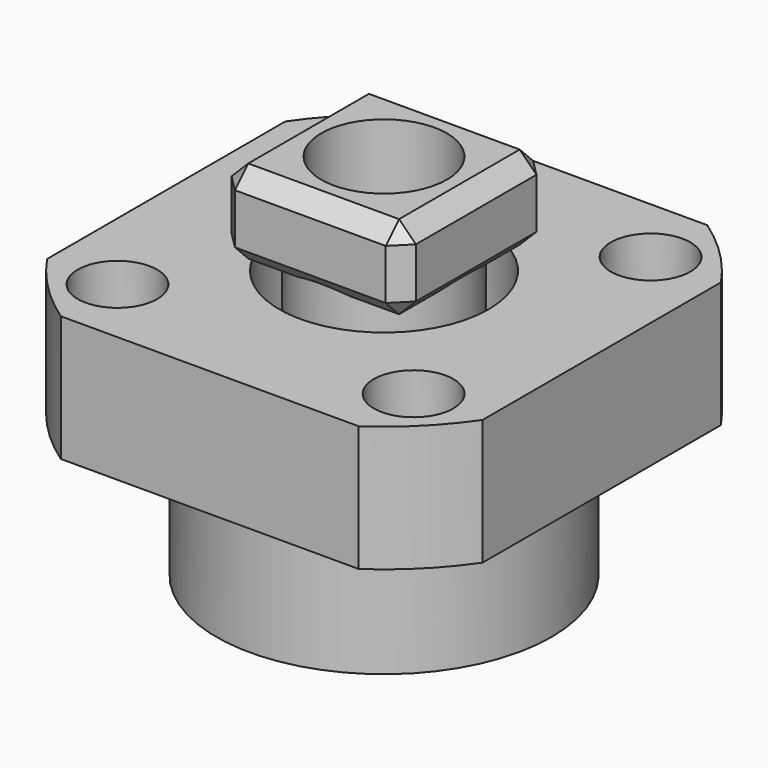
from build123d import *

# Parameters (mm, degrees)
F0_R            = 20
F1_DEPTH        = 17
F3_DEPTH        = 15
F4_R            = 12.5
F4_R_2          = 9.5
F5_DEPTH        = 10
F6_R            = 9.5
F7_DEPTH        = 2
F8_W            = 22
F8_H            = 22
F9_DEPTH        = 10
F10_T1_DEPTH    = 2.5403411844
F10_T3_DEPTH    = 2.5403411844
F10_T5_DEPTH    = 2.5403411844
F10_T7_DEPTH    = 2.5403411844
F10_T9_DEPTH    = 2.5403411844
F10_T11_DEPTH   = 2.5403411844
F10_T13_DEPTH   = 2.5403411844
F10_T15_DEPTH   = 2.5403411844
F10_T17_DEPTH   = 32.2867319519
F10_T19_DEPTH   = 32.2867319519
F10_T24_DEPTH   = 20.2867319519
F10_T29_DEPTH   = 20.2867319519
F10_T34_DEPTH   = 20.2867319519
F10_T39_DEPTH   = 20.2867319519
F10_T44_DEPTH   = 32.2867319519
F10_S45_R       = 9.5
F10_T46_DEPTH   = 18
F10_T50_DEPTH   = 32.2867319519
F10_S51_R       = 9.5
F10_T52_DEPTH   = 18
F10_T56_DEPTH   = 32.2867319519
F10_S57_R       = 9.5
F10_T58_DEPTH   = 18
F10_T62_DEPTH   = 32.2867319519
F10_S63_R       = 9.5
F10_T64_DEPTH   = 18
F11_R           = 10
F12_DEPTH       = 5
F13_R           = 7.5
F14_DEPTH       = 44.001
F16_D           = 5.5
F16_CBORE_D     = 9.5
F16_CBORE_DEPTH = 5


# Not quite as in the source:
# - a fillet or chamfer that OpenCascade refuses, or shapes differently, is made with other operations: its cross-section is extruded or revolved along the edge and cut away or added


with BuildPart() as f1:
    # F0 (on Top) → F1 (new body)
    with BuildSketch(Plane.XY):
        Circle(F0_R)
    extrude(amount=-F1_DEPTH)

    # F2 (on Top) → F3 (join)
    with BuildSketch(Plane.XY):
        with BuildLine():
            Line((17.7834192438, 26), (-17.7834192438, 26))
            ThreePointArc((-17.7834192438, 26), (-22.2738636074, 22.2738636074), (-26, 17.7834192438))
            Line((-26, 17.7834192438), (-26, -17.7834192438))
            ThreePointArc((-26, -17.7834192438), (-22.2738636074, -22.2738636074), (-17.7834192438, -26))
            Line((-17.7834192438, -26), (17.7834192438, -26))
            ThreePointArc((17.7834192438, -26), (22.2738636074, -22.2738636074), (26, -17.7834192438))
            Line((26, -17.7834192438), (26, 17.7834192438))
            ThreePointArc((26, 17.7834192438), (22.2738636074, 22.2738636074), (17.7834192438, 26))
        make_face()
    extrude(amount=F3_DEPTH)

    # F4 (on face) → F5 (cut)
    with BuildSketch(Plane.XY.offset(15)):
        Circle(F4_R)
        Circle(F4_R_2, mode=Mode.SUBTRACT)
    extrude(amount=-F5_DEPTH, mode=Mode.SUBTRACT)

    # F6 (on face) → F7 (join)
    with BuildSketch(Plane.XY.offset(15)):
        Circle(F6_R)
    extrude(amount=F7_DEPTH)

    # F8 (on face) → F9 (join)
    with BuildSketch(Plane.XY.offset(17)):
        Rectangle(F8_W, F8_H)
    extrude(amount=F9_DEPTH)

    # F10: chamfer of 2 on 12 edges, made by hand

    # F10_s2 → F10_t1 (cut)
    with BuildSketch(Plane(origin=(-0.3333333333, 0.3333333333, -0.3333333333), x_dir=(-0.7071067812, -0.7071067812, 0), z_dir=(-0.5773502692, 0.5773502692, -0.5773502692))):
        Polygon((-1.4142135624, 23.6784008469), (1.4142135624, 23.6784008469), (0, 21.2289111041), align=None)
    extrude(amount=F10_T1_DEPTH, mode=Mode.SUBTRACT)

    # F10_s4 → F10_t3 (cut)
    with BuildSketch(Plane(origin=(-15, 15, 15), x_dir=(-0.7071067812, -0.7071067812, 0), z_dir=(-0.5773502692, 0.5773502692, 0.5773502692))):
        Polygon((-1.4142135624, 12.2474487139), (1.4142135624, 12.2474487139), (0, 14.6969384567), align=None)
    extrude(amount=F10_T3_DEPTH, mode=Mode.SUBTRACT)

    # F10_s6 → F10_t5 (cut)
    with BuildSketch(Plane(origin=(0.3333333333, 0.3333333333, -0.3333333333), x_dir=(-0.7071067812, 0.7071067812, 0), z_dir=(0.5773502692, 0.5773502692, -0.5773502692))):
        Polygon((1.4142135624, 23.6784008469), (-1.4142135624, 23.6784008469), (0, 21.2289111041), align=None)
    extrude(amount=F10_T5_DEPTH, mode=Mode.SUBTRACT)

    # F10_s8 → F10_t7 (cut)
    with BuildSketch(Plane(origin=(15, 15, 15), x_dir=(-0.7071067812, 0.7071067812, 0), z_dir=(0.5773502692, 0.5773502692, 0.5773502692))):
        Polygon((1.4142135624, 12.2474487139), (-1.4142135624, 12.2474487139), (0, 14.6969384567), align=None)
    extrude(amount=F10_T7_DEPTH, mode=Mode.SUBTRACT)

    # F10_s10 → F10_t9 (cut)
    with BuildSketch(Plane(origin=(0.3333333333, -0.3333333333, -0.3333333333), x_dir=(0.7071067812, 0.7071067812, 0), z_dir=(0.5773502692, -0.5773502692, -0.5773502692))):
        Polygon((1.4142135624, 23.6784008469), (0, 21.2289111041), (-1.4142135624, 23.6784008469), align=None)
    extrude(amount=F10_T9_DEPTH, mode=Mode.SUBTRACT)

    # F10_s12 → F10_t11 (cut)
    with BuildSketch(Plane(origin=(15, -15, 15), x_dir=(0.7071067812, 0.7071067812, 0), z_dir=(0.5773502692, -0.5773502692, 0.5773502692))):
        Polygon((1.4142135624, 12.2474487139), (0, 14.6969384567), (-1.4142135624, 12.2474487139), align=None)
    extrude(amount=F10_T11_DEPTH, mode=Mode.SUBTRACT)

    # F10_s14 → F10_t13 (cut)
    with BuildSketch(Plane(origin=(-0.3333333333, -0.3333333333, -0.3333333333), x_dir=(0.7071067812, -0.7071067812, 0), z_dir=(-0.5773502692, -0.5773502692, -0.5773502692))):
        Polygon((-1.4142135624, 23.6784008469), (0, 21.2289111041), (1.4142135624, 23.6784008469), align=None)
    extrude(amount=F10_T13_DEPTH, mode=Mode.SUBTRACT)

    # F10_s16 → F10_t15 (cut)
    with BuildSketch(Plane(origin=(-15, -15, 15), x_dir=(0.7071067812, -0.7071067812, 0), z_dir=(-0.5773502692, -0.5773502692, 0.5773502692))):
        Polygon((-1.4142135624, 12.2474487139), (0, 14.6969384567), (1.4142135624, 12.2474487139), align=None)
    extrude(amount=F10_T15_DEPTH, mode=Mode.SUBTRACT)

    # F10_s18 → F10_t17 (cut)
    with BuildSketch(Plane.XZ.offset(-16.1433659759)):
        Polygon((-11, 25), (-9, 27), (-11, 27), align=None)
        Polygon((11, 25), (9, 27), (11, 27), align=None)
    extrude(amount=F10_T17_DEPTH, mode=Mode.SUBTRACT)

    # F10_s20 → F10_t19 (cut)
    with BuildSketch(Plane.YZ.offset(-16.1433659759)):
        Polygon((-9, 27), (-11, 25), (-11, 27), align=None)
        Polygon((11, 25), (9, 27), (11, 27), align=None)
    extrude(amount=F10_T19_DEPTH, mode=Mode.SUBTRACT)


with BuildPart() as f10_tool22:
    # F10_s23 → F10_t24 (new body)
    with BuildSketch(Plane.XY.offset(11.8566340241)):
        Polygon((-9, 11), (-11, 9), (-11, 11), align=None)
    extrude(amount=F10_T24_DEPTH)

    split(bisect_by=Plane.XY.offset(15), keep=Keep.TOP)


with BuildPart() as f1_1:
    add(f1.part)

    # F10_t21: cut F10_tool22
    add(f10_tool22.part, mode=Mode.SUBTRACT)


with BuildPart() as f10_tool27:
    # F10_s28 → F10_t29 (new body)
    with BuildSketch(Plane.XY.offset(11.8566340241)):
        Polygon((9, 11), (11, 9), (11, 11), align=None)
    extrude(amount=F10_T29_DEPTH)

    split(bisect_by=Plane.XY.offset(15), keep=Keep.TOP)


with BuildPart() as f1_2:
    add(f1_1.part)

    # F10_t26: cut F10_tool27
    add(f10_tool27.part, mode=Mode.SUBTRACT)


with BuildPart() as f10_tool32:
    # F10_s33 → F10_t34 (new body)
    with BuildSketch(Plane.XY.offset(11.8566340241)):
        Polygon((11, -9), (9, -11), (11, -11), align=None)
    extrude(amount=F10_T34_DEPTH)

    split(bisect_by=Plane.XY.offset(15), keep=Keep.TOP)


with BuildPart() as f1_3:
    add(f1_2.part)

    # F10_t31: cut F10_tool32
    add(f10_tool32.part, mode=Mode.SUBTRACT)


with BuildPart() as f10_tool37:
    # F10_s38 → F10_t39 (new body)
    with BuildSketch(Plane.XY.offset(11.8566340241)):
        Polygon((-11, -9), (-9, -11), (-11, -11), align=None)
    extrude(amount=F10_T39_DEPTH)

    split(bisect_by=Plane.XY.offset(15), keep=Keep.TOP)


with BuildPart() as f1_4:
    add(f1_3.part)

    # F10_t36: cut F10_tool37
    add(f10_tool37.part, mode=Mode.SUBTRACT)


with BuildPart() as f10_tool42:
    # F10_s43 → F10_t44 (new body)
    with BuildSketch(Plane.XZ.offset(-16.1433659759)):
        Polygon((-11, 19), (-9, 17), (-11, 17), align=None)
    extrude(amount=F10_T44_DEPTH)

    # F10_s45 → F10_t46 (cut, symmetric)
    with BuildSketch(Plane.XY.offset(18)):
        Circle(F10_S45_R)
    extrude(amount=F10_T46_DEPTH, both=True, mode=Mode.SUBTRACT)


with BuildPart() as f1_5:
    add(f1_4.part)

    # F10_t41: cut F10_tool42
    add(f10_tool42.part, mode=Mode.SUBTRACT)


with BuildPart() as f10_tool48:
    # F10_s49 → F10_t50 (new body)
    with BuildSketch(Plane.XZ.offset(16.1433659759)):
        Polygon((11, 19), (9, 17), (11, 17), align=None)
    extrude(amount=-F10_T50_DEPTH)

    # F10_s51 → F10_t52 (cut, symmetric)
    with BuildSketch(Plane.XY.offset(18)):
        Circle(F10_S51_R)
    extrude(amount=F10_T52_DEPTH, both=True, mode=Mode.SUBTRACT)


with BuildPart() as f1_6:
    add(f1_5.part)

    # F10_t47: cut F10_tool48
    add(f10_tool48.part, mode=Mode.SUBTRACT)


with BuildPart() as f10_tool54:
    # F10_s55 → F10_t56 (new body)
    with BuildSketch(Plane.YZ.offset(-16.1433659759)):
        Polygon((-9, 17), (-11, 19), (-11, 17), align=None)
    extrude(amount=F10_T56_DEPTH)

    # F10_s57 → F10_t58 (cut, symmetric)
    with BuildSketch(Plane.XY.offset(18)):
        Circle(F10_S57_R)
    extrude(amount=F10_T58_DEPTH, both=True, mode=Mode.SUBTRACT)


with BuildPart() as f1_7:
    add(f1_6.part)

    # F10_t53: cut F10_tool54
    add(f10_tool54.part, mode=Mode.SUBTRACT)


with BuildPart() as f10_tool60:
    # F10_s61 → F10_t62 (new body)
    with BuildSketch(Plane.YZ.offset(16.1433659759)):
        Polygon((11, 19), (9, 17), (11, 17), align=None)
    extrude(amount=-F10_T62_DEPTH)

    # F10_s63 → F10_t64 (cut, symmetric)
    with BuildSketch(Plane.XY.offset(18)):
        Circle(F10_S63_R)
    extrude(amount=F10_T64_DEPTH, both=True, mode=Mode.SUBTRACT)


with BuildPart() as f1_8:
    add(f1_7.part)

    # F10_t59: cut F10_tool60
    add(f10_tool60.part, mode=Mode.SUBTRACT)

    # F11 (on face) → F12 (cut)
    with BuildSketch(Plane(origin=(0, 0, -17), x_dir=(1, 0, 0), z_dir=(0, 0, -1))):
        Circle(F11_R)
    extrude(amount=-F12_DEPTH, mode=Mode.SUBTRACT)

    # F13 (on face) → F14 (cut, through all)
    with BuildSketch(Plane.XY.offset(27)):
        Circle(F13_R)
    extrude(amount=-F14_DEPTH, mode=Mode.SUBTRACT)

    # F16 (through all)
    with Locations(Plane.XY.offset(15)):
        with Locations((17.6776695297, 17.6776695297), (17.6776695297, -17.6776695297), (-17.6776695297, -17.6776695297), (-17.6776695297, 17.6776695297)):
            CounterBoreHole(F16_D / 2, F16_CBORE_D / 2, F16_CBORE_DEPTH)


solid = f1_8.part
